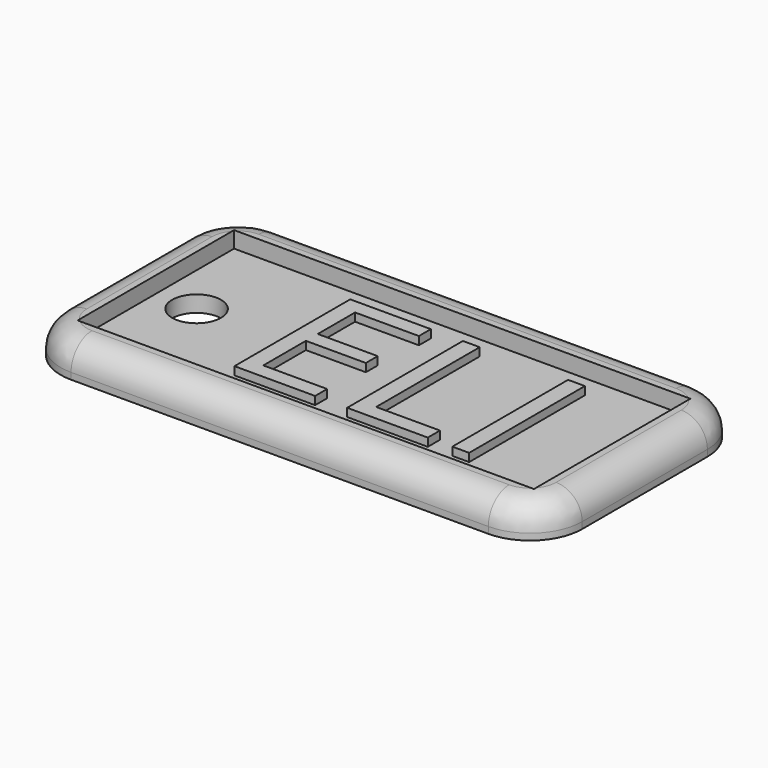
from build123d import *

# Parameters (mm, degrees)
F0_W         = 44.45
F0_H         = 19.05
F0_R         = 2.38125
F1_DEPTH     = 1.5875
F0_W_2       = 50.8
F0_H_2       = 25.4
F2_DEPTH     = 3.175
F3_R         = 5.08
F4_T1_DEPTH  = 40.64
F4_T3_DEPTH  = 15.24
F4_T6_ANGLE  = 90
F4_T8_ANGLE  = 90
F4_T10_ANGLE = 90
F4_T12_ANGLE = 90
F5_TEXT_SIZE = 19.7375296719
F6_DEPTH     = 0.79375


# Not quite as in the source:
# - a fillet or chamfer that OpenCascade refuses, or shapes differently, is made with other operations: its cross-section is extruded or revolved along the edge and cut away or added
# - Text() gives the source's letters only with a copy of the font that has no kerning and outlines rounded to 1/6400 em; it was checked with that copy


with BuildPart() as f1:
    # F0 (on Top) → F1 (new body)
    with BuildSketch(Plane.XY):
        with Locations((25.4, 12.7)):
            Rectangle(F0_W, F0_H)
        with Locations((7.14375, 12.7)):
            Circle(F0_R, mode=Mode.SUBTRACT)
    extrude(amount=F1_DEPTH)

    # F0 (on Top) → F2 (join)
    with BuildSketch(Plane.XY):
        with Locations((25.4, 12.7)):
            Rectangle(F0_W_2, F0_H_2)
        with Locations((25.4, 12.7)):
            Rectangle(F0_W, F0_H, mode=Mode.SUBTRACT)
    extrude(amount=F2_DEPTH)

    # F3
    f3_edges = [f1.edges().sort_by_distance(p)[0] for p in [
        (0, 0, 1.5875),
        (50.8, 0, 1.5875),
        (50.8, 25.4, 1.5875),
        (0, 25.4, 1.5875),
    ]]
    fillet(f3_edges, radius=F3_R)

    # F4: fillet of radius 2.54 on 8 edges, made by hand

    # F4_s2 → F4_t1 (cut)
    with BuildSketch(Plane.YZ.offset(5.08)):
        with BuildLine():
            ThreePointArc((0, 0.635), (0.7439487758, 2.4310512242), (2.54, 3.175))
            Line((2.54, 3.175), (0, 3.175))
            Line((0, 3.175), (0, 0.635))
        make_face()
        with BuildLine():
            ThreePointArc((25.4, 0.635), (24.6560512242, 2.4310512242), (22.86, 3.175))
            Line((22.86, 3.175), (25.4, 3.175))
            Line((25.4, 3.175), (25.4, 0.635))
        make_face()
    extrude(amount=F4_T1_DEPTH, mode=Mode.SUBTRACT)

    # F4_s4 → F4_t3 (cut)
    with BuildSketch(Plane.XZ.offset(-20.32)):
        with BuildLine():
            ThreePointArc((0, 0.635), (0.7439487758, 2.4310512242), (2.54, 3.175))
            Line((2.54, 3.175), (0, 3.175))
            Line((0, 3.175), (0, 0.635))
        make_face()
        with BuildLine():
            ThreePointArc((50.8, 0.635), (50.0560512242, 2.4310512242), (48.26, 3.175))
            Line((48.26, 3.175), (50.8, 3.175))
            Line((50.8, 3.175), (50.8, 0.635))
        make_face()
    extrude(amount=F4_T3_DEPTH, mode=Mode.SUBTRACT)

    # F4_s5 → F4_t6 (revolve, cut)
    with BuildSketch(Plane.XZ.offset(-20.32)):
        with BuildLine():
            ThreePointArc((0, 0.635), (0.7439487758, 2.4310512242), (2.54, 3.175))
            Line((2.54, 3.175), (0, 3.175))
            Line((0, 3.175), (0, 0.635))
        make_face()
    revolve(axis=Axis((5.08, 20.32, 3.175), (0, 0, -1)), revolution_arc=F4_T6_ANGLE, mode=Mode.SUBTRACT)

    # F4_s7 → F4_t8 (revolve, cut)
    with BuildSketch(Plane.XZ.offset(-5.08)):
        with BuildLine():
            ThreePointArc((0, 0.635), (0.7439487758, 2.4310512242), (2.54, 3.175))
            Line((2.54, 3.175), (0, 3.175))
            Line((0, 3.175), (0, 0.635))
        make_face()
    revolve(axis=Axis((5.08, 5.08, 3.175), (0, 0, 1)), revolution_arc=F4_T8_ANGLE, mode=Mode.SUBTRACT)

    # F4_s9 → F4_t10 (revolve, cut)
    with BuildSketch(Plane.XZ.offset(-20.32)):
        with BuildLine():
            ThreePointArc((50.8, 0.635), (50.0560512242, 2.4310512242), (48.26, 3.175))
            Line((48.26, 3.175), (50.8, 3.175))
            Line((50.8, 3.175), (50.8, 0.635))
        make_face()
    revolve(axis=Axis((45.72, 20.32, 3.175), (0, 0, 1)), revolution_arc=F4_T10_ANGLE, mode=Mode.SUBTRACT)

    # F4_s11 → F4_t12 (revolve, cut)
    with BuildSketch(Plane.YZ.offset(45.72)):
        with BuildLine():
            ThreePointArc((0, 0.635), (0.7439487758, 2.4310512242), (2.54, 3.175))
            Line((2.54, 3.175), (0, 3.175))
            Line((0, 3.175), (0, 0.635))
        make_face()
    revolve(axis=Axis((45.72, 5.08, 3.175), (0, 0, 1)), revolution_arc=F4_T12_ANGLE, mode=Mode.SUBTRACT)

    # F5 (on face) → F6 (join)
    with BuildSketch(Plane.XY.offset(1.5875)):
        with Locations((14.3083585426, 5.937481299)):
            Text('ELI', F5_TEXT_SIZE, font='Open Sans', text_align=(TextAlign.LEFT, TextAlign.BOTTOM))
    extrude(amount=F6_DEPTH)


solid = f1.part
